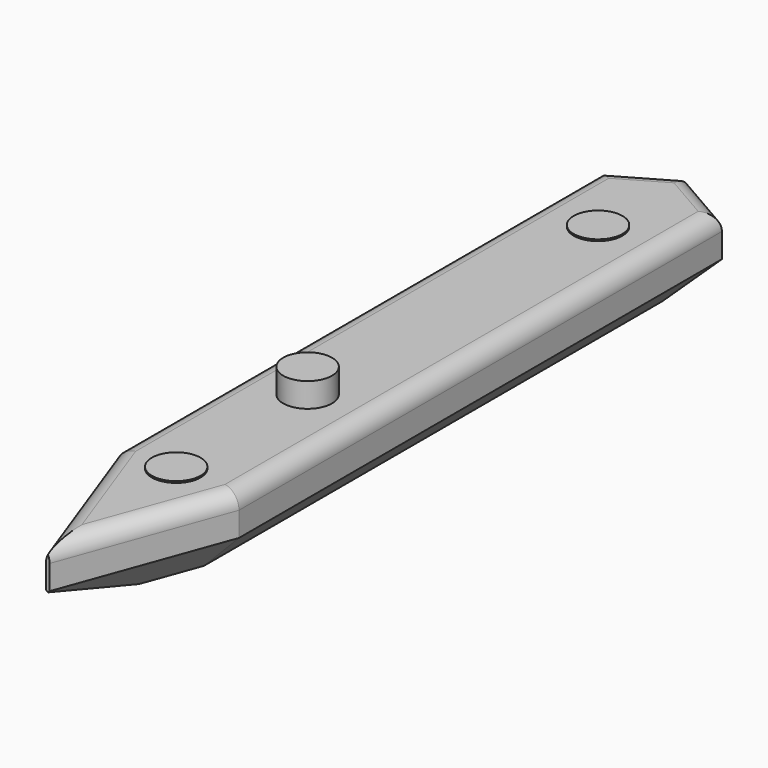
from build123d import *

# Parameters (mm, degrees)
F0_W          = 1905
F0_H          = 12700
F1_DEPTH      = 1270
F2_SIZE2      = 924.4843950362
F2_SIZE       = 2540
F2_2_SIZE2    = 924.4843950362
F2_2_SIZE     = 2540
F3_T1_DEPTH   = 7841.1978168008
F4_R          = 381
F5_DEPTH      = 381
F6_R          = 381
F7_DEPTH      = 25.4
F8_R          = 381
F9_DEPTH      = 25.4
F10_T1_DEPTH  = 7112.1620249564
F10_T3_DEPTH  = 13835.9156409968
F10_T5_DEPTH  = 4365.8896575229
F10_T7_DEPTH  = 4365.8896575229
F10_T9_DEPTH  = 7112.1620249564
F10_T14_DEPTH = 3322.0686046444
F10_T19_DEPTH = 3322.0686046444
F11_T1_DEPTH  = 11141.2651581292
F11_T3_DEPTH  = 4417.5115420888
F11_T5_DEPTH  = 4417.5115420888
F11_T7_DEPTH  = 2369.8522628062
F11_T9_DEPTH  = 2369.8522628062


# Not quite as in the source:
# - a fillet or chamfer that OpenCascade refuses, or shapes differently, is made with other operations: its cross-section is extruded or revolved along the edge and cut away or added


with BuildPart() as f1:
    # F0 (on Top) → F1 (new body)
    with BuildSketch(Plane.XY):
        Rectangle(F0_W, F0_H)
    extrude(amount=F1_DEPTH)

    # F2
    f2_edges = [f1.edges().sort_by_distance(p)[0] for p in [
        (952.5, -6350, 635),
    ]]
    f2_side = f1.faces().sort_by_distance((952.5, 0, 635))[0]
    chamfer(f2_edges, length=F2_SIZE, length2=F2_SIZE2, reference=f2_side)

    # F2#2
    f2_2_edges = [f1.edges().sort_by_distance(p)[0] for p in [
        (-952.5, -6350, 635),
    ]]
    f2_2_side = f1.faces().sort_by_distance((-952.5, 0, 635))[0]
    chamfer(f2_2_edges, length=F2_2_SIZE, length2=F2_2_SIZE2, reference=f2_2_side)

    # F3: chamfer of 1270 x 733.2348418708 on 2 edges, made by hand

    # F3_s2 → F3_t1 (cut)
    with BuildSketch(Plane.XY.offset(-3285.5989084004)):
        Polygon((952.5, 5616.7651581292), (-317.5, 6350), (952.5, 6350), align=None)
        Polygon((-952.5, 5616.7651581292), (317.5, 6350), (-952.5, 6350), align=None)
    extrude(amount=F3_T1_DEPTH, mode=Mode.SUBTRACT)

    # F4 (on face) → F5 (join)
    with BuildSketch(Plane.XY.offset(1270)):
        with Locations((0, -1280.3941220168)):
            Circle(F4_R)
    extrude(amount=F5_DEPTH)

    # F6 (on face) → F7 (join)
    with BuildSketch(Plane.XY.offset(1270)):
        with Locations((0, 4389.6043354776)):
            Circle(F6_R)
    extrude(amount=F7_DEPTH)

    # F8 (on face) → F9 (join)
    with BuildSketch(Plane.XY.offset(1270)):
        with Locations((-28.0156049638, -3810)):
            Circle(F8_R)
    extrude(amount=F9_DEPTH)

    # F10: chamfer of 635 on 7 edges, made by hand

    # F10_s2 → F10_t1 (cut)
    with BuildSketch(Plane(origin=(163.5960713175, -449.4765118562, 0), x_dir=(0, 0, 1), z_dir=(0.3420201433, -0.9396926208, 0))):
        Polygon((0, 1563.1539673694), (635, 2198.1539673694), (0, 2198.1539673694), align=None)
    extrude(amount=F10_T1_DEPTH, mode=Mode.SUBTRACT)

    # F10_s4 → F10_t3 (cut)
    with BuildSketch(Plane.XZ.offset(-7249.7838554876)):
        Polygon((-317.5, 0), (-952.5, 635), (-952.5, 0), align=None)
        Polygon((317.5, 0), (952.5, 635), (952.5, 0), align=None)
    extrude(amount=F10_T3_DEPTH, mode=Mode.SUBTRACT)

    # F10_s6 → F10_t5 (cut)
    with BuildSketch(Plane(origin=(4084.4913337829, 2358.1821710622, 0), x_dir=(0, 0, 1), z_dir=(-0.8660254038, -0.5, 0))):
        Polygon((0, 4705.5113140312), (635, 5340.5113140312), (0, 5340.5113140312), align=None)
    extrude(amount=F10_T5_DEPTH, mode=Mode.SUBTRACT)

    # F10_s8 → F10_t7 (cut)
    with BuildSketch(Plane(origin=(-4084.4913337829, 2358.1821710622, 0), x_dir=(0, 0, 1), z_dir=(0.8660254038, -0.5, 0))):
        Polygon((0, -4705.5113140312), (635, -5340.5113140312), (0, -5340.5113140312), align=None)
    extrude(amount=F10_T7_DEPTH, mode=Mode.SUBTRACT)

    # F10_s10 → F10_t9 (cut)
    with BuildSketch(Plane(origin=(-163.5960713175, -449.4765118562, 0), x_dir=(0, 0, 1), z_dir=(-0.3420201433, -0.9396926208, 0))):
        Polygon((0, -1563.1539673694), (635, -2198.1539673694), (0, -2198.1539673694), align=None)
    extrude(amount=F10_T9_DEPTH, mode=Mode.SUBTRACT)


with BuildPart() as f10_tool12:
    # F10_s13 → F10_t14 (new body)
    with BuildSketch(Plane.YZ.offset(-1661.0343023222)):
        Polygon((-6350, 635), (-5715, 0), (-6350, 0), align=None)
    extrude(amount=F10_T14_DEPTH)

    split(bisect_by=Plane(origin=(-734.4421241446, -267.3150719799, -781.5769836847), x_dir=(0.3420201433, -0.9396926208, 0), z_dir=(-0.6644630244, -0.2418447626, -0.7071067812)), keep=Keep.TOP)


with BuildPart() as f1_1:
    add(f1.part)

    # F10_t11: cut F10_tool12
    add(f10_tool12.part, mode=Mode.SUBTRACT)


with BuildPart() as f10_tool17:
    # F10_s18 → F10_t19 (new body)
    with BuildSketch(Plane.YZ.offset(-1661.0343023222)):
        Polygon((-6350, 635), (-5715, 0), (-6350, 0), align=None)
    extrude(amount=F10_T19_DEPTH)

    split(bisect_by=Plane(origin=(734.4421241446, -267.3150719799, -781.5769836847), x_dir=(0.3420201433, 0.9396926208, 0), z_dir=(0.6644630244, -0.2418447626, -0.7071067812)), keep=Keep.TOP)


with BuildPart() as f1_2:
    add(f1_1.part)

    # F10_t16: cut F10_tool17
    add(f10_tool17.part, mode=Mode.SUBTRACT)

    # F11: fillet of radius 254 on 6 edges, made by hand

    # F11_s2 → F11_t1 (cut)
    with BuildSketch(Plane.XZ.offset(-6251.7651581292)):
        with BuildLine():
            ThreePointArc((952.5, 1016), (878.1051224214, 1195.6051224214), (698.5, 1270))
            Line((698.5, 1270), (952.5, 1270))
            Line((952.5, 1270), (952.5, 1016))
        make_face()
        with BuildLine():
            ThreePointArc((-952.5, 1016), (-878.1051224214, 1195.6051224214), (-698.5, 1270))
            Line((-698.5, 1270), (-952.5, 1270))
            Line((-952.5, 1270), (-952.5, 1016))
        make_face()
    extrude(amount=F11_T1_DEPTH, mode=Mode.SUBTRACT)

    # F11_s4 → F11_t3 (cut)
    with BuildSketch(Plane(origin=(-743.8783177682, -2043.78888089, 0), x_dir=(0, 0, 1), z_dir=(-0.3420201433, -0.9396926208, 0))):
        with BuildLine():
            ThreePointArc((1270, -1944.1539673694), (1195.6051224214, -2123.7590897908), (1016, -2198.1539673694))
            Line((1016, -2198.1539673694), (1270, -2198.1539673694))
            Line((1270, -2198.1539673694), (1270, -1944.1539673694))
        make_face()
    extrude(amount=F11_T3_DEPTH, mode=Mode.SUBTRACT)

    # F11_s6 → F11_t5 (cut)
    with BuildSketch(Plane(origin=(743.8783177682, -2043.7888808901, 0), x_dir=(0, 0, 1), z_dir=(0.3420201433, -0.9396926208, 0))):
        with BuildLine():
            ThreePointArc((1016, 2198.1539673694), (1195.6051224214, 2123.7590897907), (1270, 1944.1539673694))
            Line((1270, 1944.1539673694), (1270, 2198.1539673694))
            Line((1270, 2198.1539673694), (1016, 2198.1539673694))
        make_face()
    extrude(amount=F11_T5_DEPTH, mode=Mode.SUBTRACT)

    # F11_s8 → F11_t7 (cut)
    with BuildSketch(Plane(origin=(3220.1817884187, 1859.172822383, 0), x_dir=(0, 0, 1), z_dir=(-0.8660254038, -0.5, 0))):
        with BuildLine():
            ThreePointArc((1016, 5340.5113140312), (1195.6051224214, 5266.1164364526), (1270, 5086.5113140312))
            Line((1270, 5086.5113140312), (1270, 5340.5113140312))
            Line((1270, 5340.5113140312), (1016, 5340.5113140312))
        make_face()
    extrude(amount=F11_T7_DEPTH, mode=Mode.SUBTRACT)

    # F11_s10 → F11_t9 (cut)
    with BuildSketch(Plane(origin=(-3220.1817884187, 1859.172822383, 0), x_dir=(0, 0, 1), z_dir=(0.8660254038, -0.5, 0))):
        with BuildLine():
            ThreePointArc((1016, -5340.5113140312), (1195.6051224214, -5266.1164364526), (1270, -5086.5113140312))
            Line((1270, -5086.5113140312), (1270, -5340.5113140312))
            Line((1270, -5340.5113140312), (1016, -5340.5113140312))
        make_face()
    extrude(amount=F11_T9_DEPTH, mode=Mode.SUBTRACT)


solid = f1_2.part
